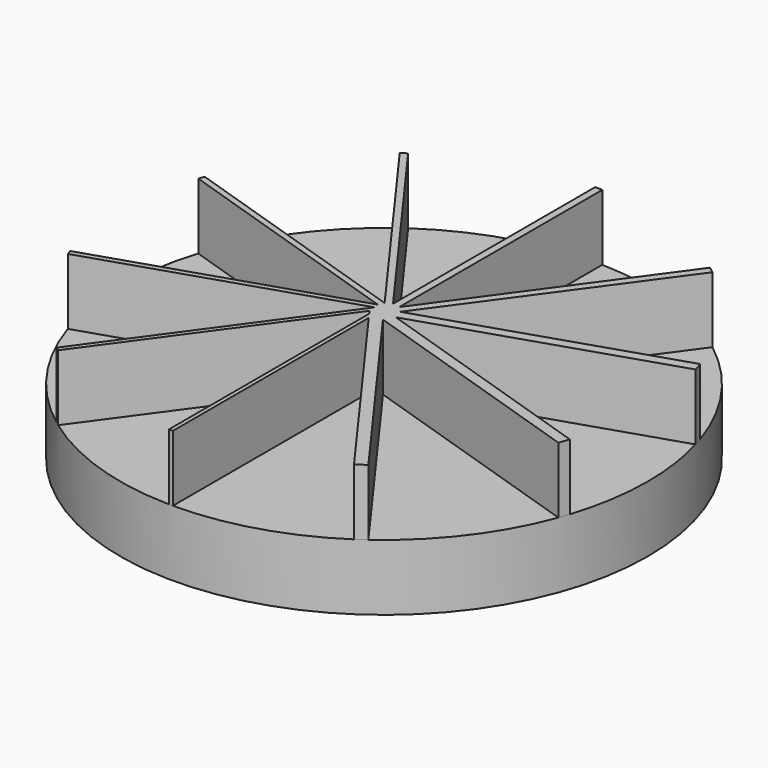
from build123d import *

# Parameters (mm, degrees)
F0_R     = 100
F1_DEPTH = 25
F3_DEPTH = 25


# Not quite as in the source:
# - a feature of the source that left no trace in its solid (it failed there, or was rolled back) is left out


with BuildPart() as f1:
    # F0 (on Top) → F1 (new body)
    with BuildSketch(Plane.XY):
        Circle(F0_R)
    extrude(amount=F1_DEPTH)

    # F2 (on face) → F3 (join)
    with BuildSketch(Plane.XY.offset(25)):
        with BuildLine():
            Line((4, -5.5055276819), (0, -4.205848897))
            Line((0, -4.205848897), (0, -7.230531871))
            Line((0, -7.230531871), (55.287094655, -83.3266893895))
            ThreePointArc((55.287094655, -83.3266893895), (57.0456970679, -82.1327489254), (58.7785252292, -80.9016994375))
            Line((58.7785252292, -80.9016994375), (4, -5.5055276819))
        make_face()
        with BuildLine():
            Line((6.0676274578, -1.9714916704), (2.3176274578, -3.1899405313))
            Line((2.3176274578, -3.1899405313), (4, -5.5055276819))
            Line((4, -5.5055276819), (93.7934686725, -34.6811942467))
            ThreePointArc((93.7934686725, -34.6811942467), (94.4684632985, -32.7980097266), (95.1056516295, -30.9016994375))
            Line((95.1056516295, -30.9016994375), (6.0676274578, -1.9714916704))
        make_face()
        with BuildLine():
            ThreePointArc((2.5, 0), (2.4692208515, -0.3910861626), (2.3776412907, -0.7725424859))
            Line((2.3776412907, -0.7725424859), (3, -0.9747590887))
            Line((3, -0.9747590887), (4.8541019662, 1.5771933364))
            Line((4.8541019662, 1.5771933364), (2.75, 0.8935291646))
            Line((2.75, 0.8935291646), (2.3776412907, 0.7725424859))
            ThreePointArc((2.3776412907, 0.7725424859), (2.4692208515, 0.3910861626), (2.5, 0))
        make_face()
        with BuildLine():
            ThreePointArc((2.0225424859, 1.4694631307), (2.2275163105, 1.1349762493), (2.3776412907, 0.7725424859))
            Line((2.3776412907, 0.7725424859), (2.75, 0.8935291646))
            Line((2.75, 0.8935291646), (2.75, 3.7850502813))
            Line((2.75, 3.7850502813), (1.5450849719, 2.1266270209))
            Line((1.5450849719, 2.1266270209), (2.0225424859, 1.4694631307))
        make_face()
        with BuildLine():
            ThreePointArc((0, 2.5), (0.7725424859, 2.3776412907), (1.4694631307, 2.0225424859))
            Line((1.4694631307, 2.0225424859), (1.5450849719, 2.1266270209))
            Line((1.5450849719, 2.1266270209), (0, 4.2532540418))
            Line((0, 4.2532540418), (0, 2.5))
        make_face()
        with BuildLine():
            ThreePointArc((-0.3411015737, 2.4766206242), (-0.1709509277, 2.4941483076), (0, 2.5))
            Line((0, 2.5), (0, 4.2532540418))
            Line((0, 4.2532540418), (-56.7376115832, 82.3458768356))
            ThreePointArc((-56.7376115832, 82.3458768356), (-57.7625819896, 81.6301667393), (-58.7785252292, 80.9016994375))
            Line((-58.7785252292, 80.9016994375), (-2.25, 3.0968593211))
            Line((-2.25, 3.0968593211), (-0.3411015737, 2.4766206242))
        make_face()
        with BuildLine():
            ThreePointArc((-2.0446187632, 1.438587541), (-1.7811355181, 1.7542965161), (-1.4694631307, 2.0225424859))
            Line((-1.4694631307, 2.0225424859), (-2.25, 3.0968593211))
            Line((-2.25, 3.0968593211), (-94.3862867265, 33.0337536163))
            ThreePointArc((-94.3862867265, 33.0337536163), (-94.7519661497, 31.9697499328), (-95.1056516295, 30.9016994375))
            Line((-95.1056516295, 30.9016994375), (-3.2360679775, 1.0514622242))
            Line((-3.2360679775, 1.0514622242), (-2.0446187632, 1.438587541))
        make_face()
        with BuildLine():
            ThreePointArc((-2.4651863178, -0.4157600492), (-2.4932429766, 0.1836830415), (-2.3776412907, 0.7725424859))
            Line((-2.3776412907, 0.7725424859), (-3.2360679775, 1.0514622242))
            Line((-3.2360679775, 1.0514622242), (-95.7046625854, -28.9934054469))
            ThreePointArc((-95.7046625854, -28.9934054469), (-95.4099282003, -29.9490500819), (-95.1056516295, -30.9016994375))
            Line((-95.1056516295, -30.9016994375), (-2.8315594803, -0.9200294462))
            Line((-2.8315594803, -0.9200294462), (-2.4651863178, -0.4157600492))
        make_face()
        with BuildLine():
            ThreePointArc((-1.5, -2), (-2.0336392212, -1.4540672329), (-2.3776412907, -0.7725424859))
            Line((-2.3776412907, -0.7725424859), (-2.8315594803, -0.9200294462))
            Line((-2.8315594803, -0.9200294462), (-60.1853038185, -79.8606862246))
            ThreePointArc((-60.1853038185, -79.8606862246), (-59.4841918711, -80.384270336), (-58.7785252292, -80.9016994375))
            Line((-58.7785252292, -80.9016994375), (-2.6266444522, -3.6152659355))
            Line((-2.6266444522, -3.6152659355), (-1.5, -2.0645728807))
            Line((-1.5, -2.0645728807), (-1.5, -2))
        make_face()
        with BuildLine():
            Line((0, -100), (0, -7.230531871))
            Line((0, -7.230531871), (-1.5, -5.1659589903))
            Line((-1.5, -5.1659589903), (-1.5, -99.9887493671))
            ThreePointArc((-1.5, -99.9887493671), (-0.7500210958, -99.9971873022), (0, -100))
        make_face()
        with BuildLine():
            Line((0, 4.2532540418), (1.5450849719, 2.1266270209))
            Line((1.5450849719, 2.1266270209), (2.75, 3.7850502813))
            Line((2.75, 3.7850502813), (2.75, 99.9621803484))
            ThreePointArc((2.75, 99.9621803484), (1.3751300235, 99.9905446401), (0, 100))
            Line((0, 100), (0, 4.2532540418))
        make_face()
        with BuildLine():
            Line((2.75, 3.7850502813), (2.75, 0.8935291646))
            Line((2.75, 0.8935291646), (4.8541019662, 1.5771933364))
            Line((4.8541019662, 1.5771933364), (61.179119922, 79.1019297209))
            ThreePointArc((61.179119922, 79.1019297209), (59.9855728515, 80.010818329), (58.7785252292, 80.9016994375))
            Line((58.7785252292, 80.9016994375), (2.75, 3.7850502813))
        make_face()
        with BuildLine():
            Line((4.8541019662, 1.5771933364), (3, -0.9747590887))
            Line((3, -0.9747590887), (6.0676274578, -1.9714916704))
            Line((6.0676274578, -1.9714916704), (96.1975706712, 27.3135020999))
            ThreePointArc((96.1975706712, 27.3135020999), (95.6684352631, 29.1127204897), (95.1056516295, 30.9016994375))
            Line((95.1056516295, 30.9016994375), (4.8541019662, 1.5771933364))
        make_face()
        with BuildLine():
            Line((1.5450849719, 2.1266270209), (1.4694631307, 2.0225424859))
            ThreePointArc((1.4694631307, 2.0225424859), (1.767766953, 1.767766953), (2.0225424859, 1.4694631307))
            Line((2.0225424859, 1.4694631307), (1.5450849719, 2.1266270209))
        make_face()
        with BuildLine():
            ThreePointArc((-1.4694631307, 2.0225424859), (-0.9333182073, 2.3192492587), (-0.3411015737, 2.4766206242))
            Line((-0.3411015737, 2.4766206242), (-2.25, 3.0968593211))
            Line((-2.25, 3.0968593211), (-1.4694631307, 2.0225424859))
        make_face()
        with BuildLine():
            ThreePointArc((-2.3776412907, 0.7725424859), (-2.2360679775, 1.1180339887), (-2.0446187632, 1.438587541))
            Line((-2.0446187632, 1.438587541), (-3.2360679775, 1.0514622242))
            Line((-3.2360679775, 1.0514622242), (-2.3776412907, 0.7725424859))
        make_face()
        with BuildLine():
            ThreePointArc((-2.3776412907, -0.7725424859), (-2.427976161, -0.5957614973), (-2.4651863178, -0.4157600492))
            Line((-2.4651863178, -0.4157600492), (-2.8315594803, -0.9200294462))
            Line((-2.8315594803, -0.9200294462), (-2.3776412907, -0.7725424859))
        make_face()
        with BuildLine():
            Line((-1.5, -2.0645728807), (-1.4694631307, -2.0225424859))
            ThreePointArc((-1.4694631307, -2.0225424859), (-1.4847743472, -2.0113291968), (-1.5, -2))
            Line((-1.5, -2), (-1.5, -2.0645728807))
        make_face()
        with BuildLine():
            ThreePointArc((1.4694631307, -2.0225424859), (0.7725424859, -2.3776412907), (0, -2.5))
            Line((0, -2.5), (0, -4.205848897))
            Line((0, -4.205848897), (4, -5.5055276819))
            Line((4, -5.5055276819), (2.3176274578, -3.1899405313))
            Line((2.3176274578, -3.1899405313), (1.4694631307, -2.0225424859))
        make_face()
        with BuildLine():
            ThreePointArc((2.3776412907, -0.7725424859), (2.0225424859, -1.4694631307), (1.4694631307, -2.0225424859))
            Line((1.4694631307, -2.0225424859), (2.3176274578, -3.1899405313))
            Line((2.3176274578, -3.1899405313), (6.0676274578, -1.9714916704))
            Line((6.0676274578, -1.9714916704), (3, -0.9747590887))
            Line((3, -0.9747590887), (2.3776412907, -0.7725424859))
        make_face()
        with BuildLine():
            Line((0, -4.205848897), (0, -2.5))
            ThreePointArc((0, -2.5), (-0.7725424859, -2.3776412907), (-1.4694631307, -2.0225424859))
            Line((-1.4694631307, -2.0225424859), (-1.5, -2.0645728807))
            Line((-1.5, -2.0645728807), (-1.5, -5.1659589903))
            Line((-1.5, -5.1659589903), (0, -7.230531871))
            Line((0, -7.230531871), (0, -4.205848897))
        make_face()
        Polygon((-1.5, -5.1659589903), (-1.5, -2.0645728807), (-2.6266444522, -3.6152659355), align=None)
        with BuildLine():
            Line((1.4694631307, -2.0225424859), (0, 0))
            Line((0, 0), (0, -2.5))
            ThreePointArc((0, -2.5), (0.7725424859, -2.3776412907), (1.4694631307, -2.0225424859))
        make_face()
        with BuildLine():
            Line((2.3776412907, -0.7725424859), (0, 0))
            Line((0, 0), (1.4694631307, -2.0225424859))
            ThreePointArc((1.4694631307, -2.0225424859), (2.0225424859, -1.4694631307), (2.3776412907, -0.7725424859))
        make_face()
        with BuildLine():
            Line((2.3776412907, 0.7725424859), (0, 0))
            Line((0, 0), (2.3776412907, -0.7725424859))
            ThreePointArc((2.3776412907, -0.7725424859), (2.4692208515, -0.3910861626), (2.5, 0))
            ThreePointArc((2.5, 0), (2.4692208515, 0.3910861626), (2.3776412907, 0.7725424859))
        make_face()
        with BuildLine():
            Line((1.4694631307, 2.0225424859), (0, 0))
            Line((0, 0), (2.3776412907, 0.7725424859))
            ThreePointArc((2.3776412907, 0.7725424859), (2.2275163105, 1.1349762493), (2.0225424859, 1.4694631307))
            ThreePointArc((2.0225424859, 1.4694631307), (1.767766953, 1.767766953), (1.4694631307, 2.0225424859))
        make_face()
        with BuildLine():
            Line((0, 2.3657900045), (0, 0))
            Line((0, 0), (1.4694631307, 2.0225424859))
            ThreePointArc((1.4694631307, 2.0225424859), (0.7725424859, 2.3776412907), (0, 2.5))
            Line((0, 2.5), (0, 2.3657900045))
        make_face()
        with BuildLine():
            Line((-1.2360679775, 1.7013016167), (0, 0))
            Line((0, 0), (0, 2.3657900045))
            Line((0, 2.3657900045), (-0.3411015737, 2.4766206242))
            ThreePointArc((-0.3411015737, 2.4766206242), (-0.9333182073, 2.3192492587), (-1.4694631307, 2.0225424859))
            Line((-1.4694631307, 2.0225424859), (-1.2360679775, 1.7013016167))
        make_face()
        with BuildLine():
            Line((-1.75, 0.5686094684), (0, 0))
            Line((0, 0), (-1.2360679775, 1.7013016167))
            Line((-1.2360679775, 1.7013016167), (-2.0446187632, 1.438587541))
            ThreePointArc((-2.0446187632, 1.438587541), (-2.2360679775, 1.1180339887), (-2.3776412907, 0.7725424859))
            Line((-2.3776412907, 0.7725424859), (-1.75, 0.5686094684))
        make_face()
        with BuildLine():
            Line((-1.5, -0.4873795443), (0, 0))
            Line((0, 0), (-1.75, 0.5686094684))
            Line((-1.75, 0.5686094684), (-2.4651863178, -0.4157600492))
            ThreePointArc((-2.4651863178, -0.4157600492), (-2.427976161, -0.5957614973), (-2.3776412907, -0.7725424859))
            Line((-2.3776412907, -0.7725424859), (-1.5, -0.4873795443))
        make_face()
        with BuildLine():
            Line((-1.4694631307, -2.0225424859), (0, 0))
            Line((0, 0), (-1.5, -0.4873795443))
            Line((-1.5, -0.4873795443), (-1.5, -2))
            ThreePointArc((-1.5, -2), (-1.4847743472, -2.0113291968), (-1.4694631307, -2.0225424859))
        make_face()
        with BuildLine():
            Line((0, -2.5), (0, 0))
            Line((0, 0), (-1.4694631307, -2.0225424859))
            ThreePointArc((-1.4694631307, -2.0225424859), (-0.7725424859, -2.3776412907), (0, -2.5))
        make_face()
        with BuildLine():
            Line((-1.5, -2), (-1.5, -0.4873795443))
            Line((-1.5, -0.4873795443), (-2.3776412907, -0.7725424859))
            ThreePointArc((-2.3776412907, -0.7725424859), (-2.0336392212, -1.4540672329), (-1.5, -2))
        make_face()
        with BuildLine():
            Line((-2.4651863178, -0.4157600492), (-1.75, 0.5686094684))
            Line((-1.75, 0.5686094684), (-2.3776412907, 0.7725424859))
            ThreePointArc((-2.3776412907, 0.7725424859), (-2.4932429766, 0.1836830415), (-2.4651863178, -0.4157600492))
        make_face()
        with BuildLine():
            Line((-2.0446187632, 1.438587541), (-1.2360679775, 1.7013016167))
            Line((-1.2360679775, 1.7013016167), (-1.4694631307, 2.0225424859))
            ThreePointArc((-1.4694631307, 2.0225424859), (-1.7811355181, 1.7542965161), (-2.0446187632, 1.438587541))
        make_face()
        with BuildLine():
            Line((-0.3411015737, 2.4766206242), (0, 2.3657900045))
            Line((0, 2.3657900045), (0, 2.5))
            ThreePointArc((0, 2.5), (-0.1709509277, 2.4941483076), (-0.3411015737, 2.4766206242))
        make_face()
    extrude(amount=F3_DEPTH)


solid = f1.part
